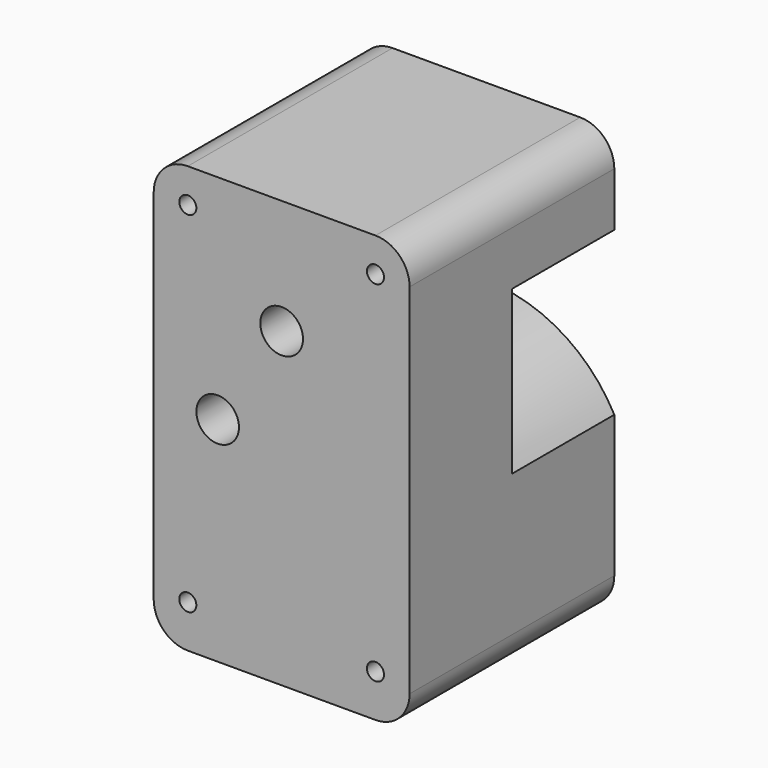
from build123d import *

# Parameters (mm, degrees)
F1_DEPTH = 38.1
F3_DEPTH = 19.05
F4_DEPTH = 38.1
F5_DEPTH = 25.4
F6_R     = 5.08
F7_R     = 3.175
F7_R_2   = 1.27
F8_DEPTH = 9.525
F9_DEPTH = 12.7
F10_R    = 5.08


# Not quite as in the source:
# - a feature names something its author has since deleted; it is built from what else it names


with BuildPart() as f1:
    # F0 (on Front) → F1 (new body)
    with BuildSketch(Plane.XZ):
        Polygon((19.05, -31.75), (19.05, 31.75), (-19.05, 31.75), (-19.05, 0), (-19.05, -31.75), align=None)
        with BuildLine():
            ThreePointArc((-6.35, 0), (-9.525, -3.175), (-12.7, 0))
            ThreePointArc((-12.7, 0), (-9.525, 3.175), (-6.35, 0))
        make_face(mode=Mode.SUBTRACT)
    extrude(amount=F1_DEPTH)

    # F2 (on face) → F3 (cut)
    with BuildSketch(Plane(origin=(0, 0, 0), x_dir=(-1, 0, 0), z_dir=(0, 1, 0))):
        with BuildLine():
            ThreePointArc((-8.89, 14.6707808959), (-6.2861792775, 20.956960188), (2.06e-08, 23.5607808959))
            ThreePointArc((2.06e-08, 23.5607808959), (-9.8358430758, 22.3144881592), (-19.05, 18.654383355))
            Line((-19.05, 18.654383355), (-19.05, 14.6707808959))
            Line((-19.05, 14.6707808959), (-8.89, 14.6707808959))
        make_face()
        with BuildLine():
            ThreePointArc((1.27, 14.6707808959), (0.8980256121, 15.5688065081), (0, 15.9407808959))
            Line((0, 15.9407808959), (0, 14.6707808959))
            Line((0, 14.6707808959), (1.27, 14.6707808959))
        make_face()
        with BuildLine():
            ThreePointArc((0, 13.4007808959), (0.8980256121, 13.7727552838), (1.27, 14.6707808959))
            Line((1.27, 14.6707808959), (0, 14.6707808959))
            Line((0, 14.6707808959), (0, 13.4007808959))
        make_face()
        with BuildLine():
            Line((0, 14.6707808959), (0, 15.9407808959))
            ThreePointArc((0, 15.9407808959), (-0.8980256121, 15.5688065081), (-1.27, 14.6707808959))
            Line((-1.27, 14.6707808959), (0, 14.6707808959))
        make_face()
        with BuildLine():
            Line((0, 14.6707808959), (-1.27, 14.6707808959))
            ThreePointArc((-1.27, 14.6707808959), (-0.8980256121, 13.7727552838), (0, 13.4007808959))
            Line((0, 13.4007808959), (0, 14.6707808959))
        make_face()
        with BuildLine():
            ThreePointArc((-1.6e-09, 5.7807808959), (-6.2861792853, 8.3846016118), (-8.89, 14.6707808959))
            Line((-8.89, 14.6707808959), (-19.05, 14.6707808959))
            Line((-19.05, 14.6707808959), (-19.05, -5.5759541115))
            ThreePointArc((-19.05, -5.5759541115), (-11.0891605869, 2.7261656541), (-1.6e-09, 5.7807808959))
        make_face()
        with BuildLine():
            Line((-1.27, 14.6707808959), (-8.89, 14.6707808959))
            ThreePointArc((-8.89, 14.6707808959), (-6.2861792853, 8.3846016118), (-1.6e-09, 5.7807808959))
            Line((0, 5.7807808959), (0, 6.7332808959))
            Line((0, 6.7332808959), (0, 13.4007808959))
            ThreePointArc((0, 13.4007808959), (-0.8980256121, 13.7727552838), (-1.27, 14.6707808959))
        make_face()
        with BuildLine():
            ThreePointArc((-1.6e-09, 5.7807808959), (6.2861792842, 8.3846016106), (8.89, 14.6707808959))
            Line((8.89, 14.6707808959), (1.27, 14.6707808959))
            ThreePointArc((1.27, 14.6707808959), (0.8980256121, 13.7727552838), (0, 13.4007808959))
            Line((0, 13.4007808959), (0, 6.7332808959))
            Line((0, 6.7332808959), (0, 5.7807808959))
        make_face()
        with BuildLine():
            ThreePointArc((8.89, 14.6707808959), (6.286179292, 20.9569601734), (2.06e-08, 23.5607808959))
            Line((0, 23.5607808959), (0, 22.6082808959))
            Line((0, 22.6082808959), (0, 15.9407808959))
            ThreePointArc((0, 15.9407808959), (0.8980256121, 15.5688065081), (1.27, 14.6707808959))
            Line((1.27, 14.6707808959), (8.89, 14.6707808959))
        make_face()
        with BuildLine():
            Line((0, 22.6082808959), (0, 23.5607808959))
            ThreePointArc((2.06e-08, 23.5607808959), (-6.2861792775, 20.956960188), (-8.89, 14.6707808959))
            Line((-8.89, 14.6707808959), (-1.27, 14.6707808959))
            ThreePointArc((-1.27, 14.6707808959), (-0.8980256121, 15.5688065081), (0, 15.9407808959))
            Line((0, 15.9407808959), (0, 22.6082808959))
        make_face()
    extrude(amount=-F3_DEPTH, mode=Mode.SUBTRACT)

    # F2 (on face) → F4 (cut)
    with BuildSketch(Plane(origin=(0, 0, 0), x_dir=(-1, 0, 0), z_dir=(0, 1, 0))):
        with BuildLine():
            Line((0, 14.6707808959), (0, 15.9407808959))
            ThreePointArc((0, 15.9407808959), (-0.8980256121, 15.5688065081), (-1.27, 14.6707808959))
            Line((-1.27, 14.6707808959), (0, 14.6707808959))
        make_face()
        with BuildLine():
            ThreePointArc((1.27, 14.6707808959), (0.8980256121, 15.5688065081), (0, 15.9407808959))
            Line((0, 15.9407808959), (0, 14.6707808959))
            Line((0, 14.6707808959), (1.27, 14.6707808959))
        make_face()
        with BuildLine():
            ThreePointArc((0, 13.4007808959), (0.8980256121, 13.7727552838), (1.27, 14.6707808959))
            Line((1.27, 14.6707808959), (0, 14.6707808959))
            Line((0, 14.6707808959), (0, 13.4007808959))
        make_face()
        with BuildLine():
            Line((0, 14.6707808959), (-1.27, 14.6707808959))
            ThreePointArc((-1.27, 14.6707808959), (-0.8980256121, 13.7727552838), (0, 13.4007808959))
            Line((0, 13.4007808959), (0, 14.6707808959))
        make_face()
    extrude(amount=-F4_DEPTH, mode=Mode.SUBTRACT)

    # F2 (on face) → F5 (cut)
    with BuildSketch(Plane(origin=(0, 0, 0), x_dir=(-1, 0, 0), z_dir=(0, 1, 0))):
        with BuildLine():
            ThreePointArc((12.7, -15.875), (8.9802561211, -6.8947438789), (0, -3.175))
            ThreePointArc((0, -3.175), (-8.9802561211, -6.8947438789), (-12.7, -15.875))
            ThreePointArc((-12.7, -15.875), (-8.9802561211, -24.8552561211), (0, -28.575))
            ThreePointArc((0, -28.575), (8.9802561211, -24.8552561211), (12.7, -15.875))
        make_face()
    extrude(amount=-F5_DEPTH, mode=Mode.SUBTRACT)

    # F6
    f6_edges = [f1.edges().sort_by_distance(p)[0] for p in [
        (19.05, -19.05, 31.75),
        (-19.05, -19.05, 31.75),
    ]]
    fillet(f6_edges, radius=F6_R)

    # F7 (on face) → F8 (cut)
    with BuildSketch(Plane.XZ.offset(38.1)):
        with BuildLine():
            Line((-13.97, 25.4), (-13.97, 26.67))
            Line((-13.97, 26.67), (-12.7, 26.67))
            ThreePointArc((-12.7, 26.67), (-14.8680256121, 27.5680256121), (-13.97, 25.4))
        make_face()
        with BuildLine():
            Line((-12.7, 26.67), (-13.97, 26.67))
            Line((-13.97, 26.67), (-13.97, 25.4))
            ThreePointArc((-13.97, 25.4), (-13.0719743879, 25.7719743879), (-12.7, 26.67))
        make_face()
        with BuildLine():
            Line((13.97, 26.67), (12.7, 26.67))
            ThreePointArc((12.7, 26.67), (13.0719743879, 25.7719743879), (13.97, 25.4))
            Line((13.97, 25.4), (13.97, 26.67))
        make_face()
        with BuildLine():
            ThreePointArc((15.24, 26.67), (13.97, 27.94), (12.7, 26.67))
            Line((12.7, 26.67), (13.97, 26.67))
            Line((13.97, 26.67), (13.97, 25.4))
            ThreePointArc((13.97, 25.4), (14.8680256121, 25.7719743879), (15.24, 26.67))
        make_face()
        with BuildLine():
            Line((-13.97, -25.4), (-13.97, -24.13))
            ThreePointArc((-13.97, -24.13), (-15.24, -25.4), (-13.97, -26.67))
            Line((-13.97, -26.67), (-13.97, -25.4))
        make_face()
        with BuildLine():
            ThreePointArc((-12.7, -25.4), (-13.0719743879, -24.5019743879), (-13.97, -24.13))
            Line((-13.97, -24.13), (-13.97, -25.4))
            Line((-13.97, -25.4), (-12.7, -25.4))
        make_face()
        with BuildLine():
            ThreePointArc((15.24, -25.4), (14.8680256121, -24.5019743879), (13.97, -24.13))
            Line((13.97, -24.13), (13.97, -25.4))
            Line((13.97, -25.4), (13.97, -26.67))
            ThreePointArc((13.97, -26.67), (14.8680256121, -26.2980256121), (15.24, -25.4))
        make_face()
        with BuildLine():
            Line((13.97, -25.4), (13.97, -24.13))
            ThreePointArc((13.97, -24.13), (13.0719743879, -24.5019743879), (12.7, -25.4))
            Line((12.7, -25.4), (13.97, -25.4))
        make_face()
        with BuildLine():
            Line((13.97, -25.4), (12.7, -25.4))
            ThreePointArc((12.7, -25.4), (13.0719743879, -26.2980256121), (13.97, -26.67))
            Line((13.97, -26.67), (13.97, -25.4))
        make_face()
        with BuildLine():
            Line((-12.7, -25.4), (-13.97, -25.4))
            Line((-13.97, -25.4), (-13.97, -26.67))
            ThreePointArc((-13.97, -26.67), (-13.0719743879, -26.2980256121), (-12.7, -25.4))
        make_face()
        with Locations((0, 14.6707808959)):
            Circle(F7_R)
        with Locations((0, 14.6707808959)):
            Circle(F7_R_2, mode=Mode.SUBTRACT)
    extrude(amount=-F8_DEPTH, mode=Mode.SUBTRACT)

    # F7 (on face) → F9 (cut)
    with BuildSketch(Plane.XZ.offset(38.1)):
        with BuildLine():
            Line((-12.7, 26.67), (-13.97, 26.67))
            Line((-13.97, 26.67), (-13.97, 25.4))
            ThreePointArc((-13.97, 25.4), (-13.0719743879, 25.7719743879), (-12.7, 26.67))
        make_face()
        with BuildLine():
            Line((-13.97, 25.4), (-13.97, 26.67))
            Line((-13.97, 26.67), (-12.7, 26.67))
            ThreePointArc((-12.7, 26.67), (-14.8680256121, 27.5680256121), (-13.97, 25.4))
        make_face()
        with BuildLine():
            Line((13.97, 26.67), (12.7, 26.67))
            ThreePointArc((12.7, 26.67), (13.0719743879, 25.7719743879), (13.97, 25.4))
            Line((13.97, 25.4), (13.97, 26.67))
        make_face()
        with BuildLine():
            ThreePointArc((15.24, 26.67), (13.97, 27.94), (12.7, 26.67))
            Line((12.7, 26.67), (13.97, 26.67))
            Line((13.97, 26.67), (13.97, 25.4))
            ThreePointArc((13.97, 25.4), (14.8680256121, 25.7719743879), (15.24, 26.67))
        make_face()
        with BuildLine():
            ThreePointArc((15.24, -25.4), (14.8680256121, -24.5019743879), (13.97, -24.13))
            Line((13.97, -24.13), (13.97, -25.4))
            Line((13.97, -25.4), (13.97, -26.67))
            ThreePointArc((13.97, -26.67), (14.8680256121, -26.2980256121), (15.24, -25.4))
        make_face()
        with BuildLine():
            Line((13.97, -25.4), (13.97, -24.13))
            ThreePointArc((13.97, -24.13), (13.0719743879, -24.5019743879), (12.7, -25.4))
            Line((12.7, -25.4), (13.97, -25.4))
        make_face()
        with BuildLine():
            Line((13.97, -25.4), (12.7, -25.4))
            ThreePointArc((12.7, -25.4), (13.0719743879, -26.2980256121), (13.97, -26.67))
            Line((13.97, -26.67), (13.97, -25.4))
        make_face()
        with BuildLine():
            Line((-12.7, -25.4), (-13.97, -25.4))
            Line((-13.97, -25.4), (-13.97, -26.67))
            ThreePointArc((-13.97, -26.67), (-13.0719743879, -26.2980256121), (-12.7, -25.4))
        make_face()
        with BuildLine():
            ThreePointArc((-12.7, -25.4), (-13.0719743879, -24.5019743879), (-13.97, -24.13))
            Line((-13.97, -24.13), (-13.97, -25.4))
            Line((-13.97, -25.4), (-12.7, -25.4))
        make_face()
        with BuildLine():
            Line((-13.97, -25.4), (-13.97, -24.13))
            ThreePointArc((-13.97, -24.13), (-15.24, -25.4), (-13.97, -26.67))
            Line((-13.97, -26.67), (-13.97, -25.4))
        make_face()
    extrude(amount=-F9_DEPTH, mode=Mode.SUBTRACT)

    # F10
    f10_edges = [f1.edges().sort_by_distance(p)[0] for p in [
        (19.05, -19.05, -31.75),
        (-19.05, -19.05, -31.75),
    ]]
    fillet(f10_edges, radius=F10_R)


solid = f1.part
